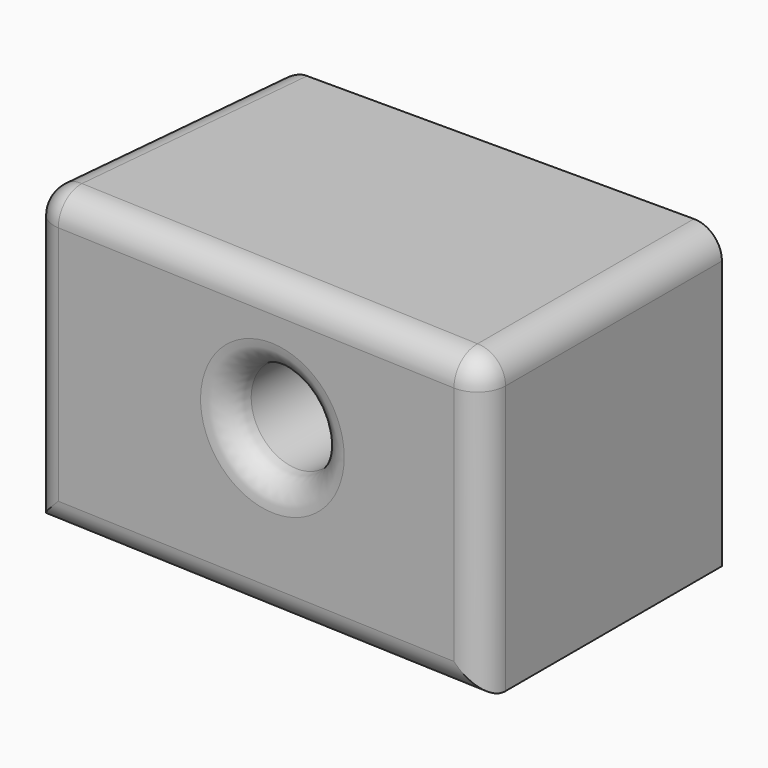
from build123d import *

# Parameters (mm, degrees)
F1_DEPTH = 53.848
F2_R     = 8.4604896976
F3_DEPTH = 64.262
F4_R     = 5.08


with BuildPart() as f1:
    # F0 (on Top) → F1 (new body)
    with BuildSketch(Plane.XY):
        Polygon((24.7506033629, 22.1318155527), (-55.6636229157, 22.1318155527), (-60.4034848511, -28.4259710461), (24.7506033629, -32.2828106582), align=None)
    extrude(amount=F1_DEPTH)

    # F2 (on face) → F3 (cut)
    with BuildSketch(Plane(origin=(-1.4085054524, -31.0979998146, 0), x_dir=(0.9989758712, -0.045246092, 0), z_dir=(-0.045246092, -0.9989758712, 0))):
        with Locations((-13.3521184325, 30.6290015578)):
            Circle(F2_R)
    extrude(amount=-F3_DEPTH, mode=Mode.SUBTRACT)

    # F4
    f4_edges = [f1.edges().sort_by_distance(p)[0] for p in [
        (-60.403485, -28.425971, 26.924),
        (-17.826441, -30.354391, 0),
        (-17.826441, -30.354391, 53.848),
        (24.750603, -32.282811, 26.924),
        (-23.198775, -30.111065, 30.629002),
        (-58.033554, -3.147078, 53.848),
        (-55.663623, 22.131816, 26.924),
        (24.750603, -5.075498, 53.848),
    ]]
    fillet(f4_edges, radius=F4_R)


solid = f1.part
